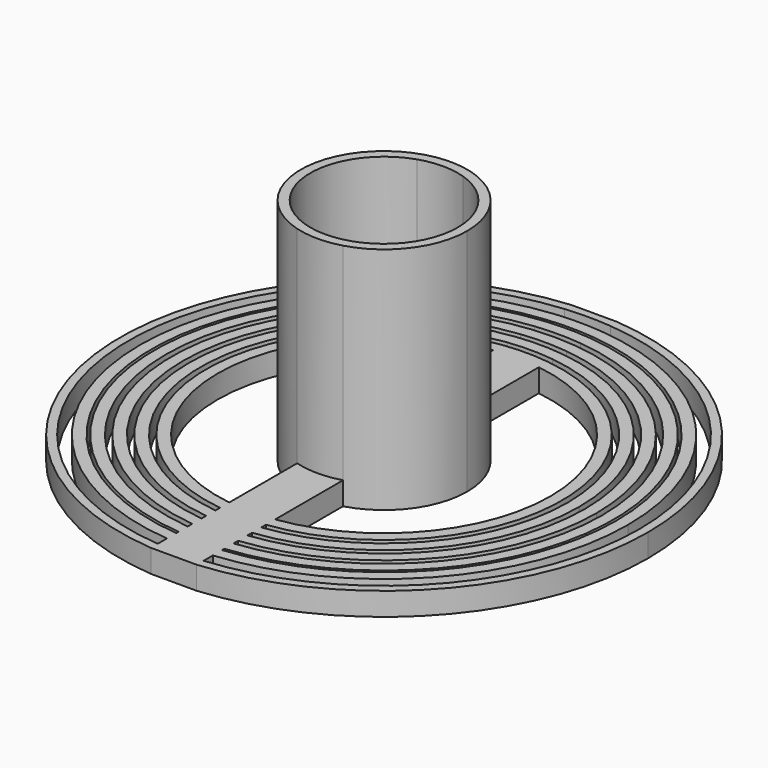
from build123d import *

# Parameters (mm, degrees)
F1_DEPTH = 40
F2_DEPTH = 4


with BuildPart() as f1:
    # F0 (on Top) → F1 (new body)
    with BuildSketch(Plane.XY):
        with BuildLine():
            ThreePointArc((4, 12.2115723803), (10.4048666498, 7.5406398933), (12.85, 0))
            ThreePointArc((12.85, 0), (10.4048666498, -7.5406398933), (4, -12.2115723803))
            Line((4, -12.2115723803), (4, -13.9373598648))
            ThreePointArc((4, -13.9373598648), (11.5812348219, -8.7249641833), (14.5, 0))
            ThreePointArc((14.5, 0), (11.5812348219, 8.7249641833), (4, 13.9373598648))
            Line((4, 13.9373598648), (4, 12.2115723803))
        make_face()
        with BuildLine():
            ThreePointArc((-4, 12.2115723803), (0, 12.85), (4, 12.2115723803))
            Line((4, 12.2115723803), (4, 13.9373598648))
            ThreePointArc((4, 13.9373598648), (0, 14.5), (-4, 13.9373598648))
            Line((-4, 13.9373598648), (-4, 12.2115723803))
        make_face()
        with BuildLine():
            Line((4, -13.9373598648), (4, -12.2115723803))
            ThreePointArc((4, -12.2115723803), (0, -12.85), (-4, -12.2115723803))
            Line((-4, -12.2115723803), (-4, -13.9373598648))
            ThreePointArc((-4, -13.9373598648), (0, -14.5), (4, -13.9373598648))
        make_face()
        with BuildLine():
            ThreePointArc((-4, -12.2115723803), (-12.85, 0), (-4, 12.2115723803))
            Line((-4, 12.2115723803), (-4, 13.9373598648))
            ThreePointArc((-4, 13.9373598648), (-14.5, 0), (-4, -13.9373598648))
            Line((-4, -13.9373598648), (-4, -12.2115723803))
        make_face()
    extrude(amount=F1_DEPTH)

    # F0 (on Top) → F2 (join)
    with BuildSketch(Plane.XY):
        with BuildLine():
            Line((4, -28.7228132327), (4, -13.9373598648))
            ThreePointArc((4, -13.9373598648), (0, -14.5), (-4, -13.9373598648))
            Line((-4, -13.9373598648), (-4, -28.7228132327))
            ThreePointArc((-4, -28.7228132327), (0, -29), (4, -28.7228132327))
        make_face()
        with BuildLine():
            ThreePointArc((-4, 40.3019850628), (0, 40.5), (4, 40.3019850628))
            Line((4, 40.3019850628), (4, 42.3113459961))
            ThreePointArc((4, 42.3113459961), (0, 42.5), (-4, 42.3113459961))
            Line((-4, 42.3113459961), (-4, 40.3019850628))
        make_face()
        with BuildLine():
            ThreePointArc((-4, -40.3019850628), (-40.5, 0), (-4, 40.3019850628))
            Line((-4, 40.3019850628), (-4, 42.3113459961))
            ThreePointArc((-4, 42.3113459961), (-42.5, 0), (-4, -42.3113459961))
            Line((-4, -42.3113459961), (-4, -40.3019850628))
        make_face()
        with BuildLine():
            Line((4, -42.3113459961), (4, -40.3019850628))
            ThreePointArc((4, -40.3019850628), (0, -40.5), (-4, -40.3019850628))
            Line((-4, -40.3019850628), (-4, -42.3113459961))
            ThreePointArc((-4, -42.3113459961), (0, -42.5), (4, -42.3113459961))
        make_face()
        with BuildLine():
            Line((4, 42.3113459961), (4, 40.3019850628))
            ThreePointArc((4, 40.3019850628), (30.0187441443, 27.1868534406), (40.5, 0))
            ThreePointArc((40.5, 0), (30.0187441443, -27.1868534406), (4, -40.3019850628))
            Line((4, -40.3019850628), (4, -42.3113459961))
            ThreePointArc((4, -42.3113459961), (31.434455618, -28.6028844699), (42.5, 0))
            ThreePointArc((42.5, 0), (31.434455618, 28.6028844699), (4, 42.3113459961))
        make_face()
        with BuildLine():
            ThreePointArc((-4, 37.7888872554), (0, 38), (4, 37.7888872554))
            Line((4, 37.7888872554), (4, 39.7994974843))
            ThreePointArc((4, 39.7994974843), (0, 40), (-4, 39.7994974843))
            Line((-4, 39.7994974843), (-4, 37.7888872554))
        make_face()
        with BuildLine():
            ThreePointArc((-4, -37.7888872554), (-38, 0), (-4, 37.7888872554))
            Line((-4, 37.7888872554), (-4, 39.7994974843))
            ThreePointArc((-4, 39.7994974843), (-40, 0), (-4, -39.7994974843))
            Line((-4, -39.7994974843), (-4, -37.7888872554))
        make_face()
        with BuildLine():
            Line((4, -39.7994974843), (4, -37.7888872554))
            ThreePointArc((4, -37.7888872554), (0, -38), (-4, -37.7888872554))
            Line((-4, -37.7888872554), (-4, -39.7994974843))
            ThreePointArc((-4, -39.7994974843), (0, -40), (4, -39.7994974843))
        make_face()
        with BuildLine():
            Line((4, 39.7994974843), (4, 37.7888872554))
            ThreePointArc((4, 37.7888872554), (28.2488937837, 25.4165300543), (38, 0))
            ThreePointArc((38, 0), (28.2488937837, -25.4165300543), (4, -37.7888872554))
            Line((4, -37.7888872554), (4, -39.7994974843))
            ThreePointArc((4, -39.7994974843), (29.6647939484, -26.83281573), (40, 0))
            ThreePointArc((40, 0), (29.6647939484, 26.83281573), (4, 39.7994974843))
        make_face()
        with BuildLine():
            Line((4, -40.3019850628), (4, -39.7994974843))
            ThreePointArc((4, -39.7994974843), (0, -40), (-4, -39.7994974843))
            Line((-4, -39.7994974843), (-4, -40.3019850628))
            ThreePointArc((-4, -40.3019850628), (0, -40.5), (4, -40.3019850628))
        make_face()
        with BuildLine():
            Line((4, -44.3198601081), (4, -42.3113459961))
            ThreePointArc((4, -42.3113459961), (0, -42.5), (-4, -42.3113459961))
            Line((-4, -42.3113459961), (-4, -44.3198601081))
            ThreePointArc((-4, -44.3198601081), (0, -44.5), (4, -44.3198601081))
        make_face()
        with BuildLine():
            ThreePointArc((-4, -44.3198601081), (-44.5, 0), (-4, 44.3198601081))
            Line((-4, 44.3198601081), (-4, 45.8257569496))
            ThreePointArc((-4, 45.8257569496), (-46, 0), (-4, -45.8257569496))
            Line((-4, -45.8257569496), (-4, -44.3198601081))
        make_face()
        with BuildLine():
            Line((4, 45.8257569496), (4, 44.3198601081))
            ThreePointArc((4, 44.3198601081), (32.8500380517, 30.0187441443), (44.5, 0))
            ThreePointArc((44.5, 0), (32.8500380517, -30.0187441443), (4, -44.3198601081))
            Line((4, -44.3198601081), (4, -45.8257569496))
            ThreePointArc((4, -45.8257569496), (33.9116499156, -31.0805405358), (46, 0))
            ThreePointArc((46, 0), (33.9116499156, 31.0805405358), (4, 45.8257569496))
        make_face()
        with BuildLine():
            ThreePointArc((-4, 44.3198601081), (0, 44.5), (4, 44.3198601081))
            Line((4, 44.3198601081), (4, 45.8257569496))
            Line((4, 45.8257569496), (-4, 45.8257569496))
            Line((-4, 45.8257569496), (-4, 44.3198601081))
        make_face()
        with BuildLine():
            Line((4, -45.8257569496), (4, -44.3198601081))
            ThreePointArc((4, -44.3198601081), (0, -44.5), (-4, -44.3198601081))
            Line((-4, -44.3198601081), (-4, -45.8257569496))
            Line((-4, -45.8257569496), (4, -45.8257569496))
        make_face()
        with BuildLine():
            ThreePointArc((-4, -34.7706773014), (-35, 0), (-4, 34.7706773014))
            Line((-4, 34.7706773014), (-4, 36.7831483155))
            ThreePointArc((-4, 36.7831483155), (-37, 0), (-4, -36.7831483155))
            Line((-4, -36.7831483155), (-4, -34.7706773014))
        make_face()
        with BuildLine():
            ThreePointArc((-4, -31.7490157328), (-32, 0), (-4, 31.7490157328))
            Line((-4, 31.7490157328), (-4, 33.7638860323))
            ThreePointArc((-4, 33.7638860323), (-34, 0), (-4, -33.7638860323))
            Line((-4, -33.7638860323), (-4, -31.7490157328))
        make_face()
        with BuildLine():
            ThreePointArc((-4, -28.7228132327), (-29, 0), (-4, 28.7228132327))
            Line((-4, 28.7228132327), (-4, 30.7408522979))
            ThreePointArc((-4, 30.7408522979), (-31, 0), (-4, -30.7408522979))
            Line((-4, -30.7408522979), (-4, -28.7228132327))
        make_face()
        with BuildLine():
            Line((4, 36.7831483155), (4, 34.7706773014))
            ThreePointArc((4, 34.7706773014), (26.1247009552, 23.2916293977), (35, 0))
            ThreePointArc((35, 0), (26.1247009552, -23.2916293977), (4, -34.7706773014))
            Line((4, -34.7706773014), (4, -36.7831483155))
            ThreePointArc((4, -36.7831483155), (27.5408787078, -24.7082982012), (37, 0))
            ThreePointArc((37, 0), (27.5408787078, 24.7082982012), (4, 36.7831483155))
        make_face()
        with BuildLine():
            Line((4, 33.7638860323), (4, 31.7490157328))
            ThreePointArc((4, 31.7490157328), (24, 21.1660104885), (32, 0))
            ThreePointArc((32, 0), (24, -21.1660104885), (4, -31.7490157328))
            Line((4, -31.7490157328), (4, -33.7638860323))
            ThreePointArc((4, -33.7638860323), (25.4165300543, -22.5831795813), (34, 0))
            ThreePointArc((34, 0), (25.4165300543, 22.5831795813), (4, 33.7638860323))
        make_face()
        with BuildLine():
            Line((4, 30.7408522979), (4, 28.7228132327))
            ThreePointArc((4, 28.7228132327), (21.8746428542, 19.0394327647), (29, 0))
            ThreePointArc((29, 0), (21.8746428542, -19.0394327647), (4, -28.7228132327))
            Line((4, -28.7228132327), (4, -30.7408522979))
            ThreePointArc((4, -30.7408522979), (23.2916293977, -20.4572725455), (31, 0))
            ThreePointArc((31, 0), (23.2916293977, 20.4572725455), (4, 30.7408522979))
        make_face()
        with BuildLine():
            ThreePointArc((-4, 28.7228132327), (0, 29), (4, 28.7228132327))
            Line((4, 28.7228132327), (4, 30.7408522979))
            ThreePointArc((4, 30.7408522979), (0, 31), (-4, 30.7408522979))
            Line((-4, 30.7408522979), (-4, 28.7228132327))
        make_face()
        with BuildLine():
            ThreePointArc((-4, 31.7490157328), (0, 32), (4, 31.7490157328))
            Line((4, 31.7490157328), (4, 33.7638860323))
            ThreePointArc((4, 33.7638860323), (0, 34), (-4, 33.7638860323))
            Line((-4, 33.7638860323), (-4, 31.7490157328))
        make_face()
        with BuildLine():
            ThreePointArc((-4, 34.7706773014), (0, 35), (4, 34.7706773014))
            Line((4, 34.7706773014), (4, 36.7831483155))
            ThreePointArc((4, 36.7831483155), (0, 37), (-4, 36.7831483155))
            Line((-4, 36.7831483155), (-4, 34.7706773014))
        make_face()
        with BuildLine():
            Line((4, -30.7408522979), (4, -28.7228132327))
            ThreePointArc((4, -28.7228132327), (0, -29), (-4, -28.7228132327))
            Line((-4, -28.7228132327), (-4, -30.7408522979))
            ThreePointArc((-4, -30.7408522979), (0, -31), (4, -30.7408522979))
        make_face()
        with BuildLine():
            Line((4, -33.7638860323), (4, -31.7490157328))
            ThreePointArc((4, -31.7490157328), (0, -32), (-4, -31.7490157328))
            Line((-4, -31.7490157328), (-4, -33.7638860323))
            ThreePointArc((-4, -33.7638860323), (0, -34), (4, -33.7638860323))
        make_face()
        with BuildLine():
            Line((4, -36.7831483155), (4, -34.7706773014))
            ThreePointArc((4, -34.7706773014), (0, -35), (-4, -34.7706773014))
            Line((-4, -34.7706773014), (-4, -36.7831483155))
            ThreePointArc((-4, -36.7831483155), (0, -37), (4, -36.7831483155))
        make_face()
        with BuildLine():
            Line((4, -31.7490157328), (4, -30.7408522979))
            ThreePointArc((4, -30.7408522979), (0, -31), (-4, -30.7408522979))
            Line((-4, -30.7408522979), (-4, -31.7490157328))
            ThreePointArc((-4, -31.7490157328), (0, -32), (4, -31.7490157328))
        make_face()
        with BuildLine():
            Line((4, -34.7706773014), (4, -33.7638860323))
            ThreePointArc((4, -33.7638860323), (0, -34), (-4, -33.7638860323))
            Line((-4, -33.7638860323), (-4, -34.7706773014))
            ThreePointArc((-4, -34.7706773014), (0, -35), (4, -34.7706773014))
        make_face()
        with BuildLine():
            Line((4, -37.7888872554), (4, -36.7831483155))
            ThreePointArc((4, -36.7831483155), (0, -37), (-4, -36.7831483155))
            Line((-4, -36.7831483155), (-4, -37.7888872554))
            ThreePointArc((-4, -37.7888872554), (0, -38), (4, -37.7888872554))
        make_face()
        with BuildLine():
            ThreePointArc((-4, 13.9373598648), (0, 14.5), (4, 13.9373598648))
            Line((4, 13.9373598648), (4, 28.7228132327))
            ThreePointArc((4, 28.7228132327), (0, 29), (-4, 28.7228132327))
            Line((-4, 28.7228132327), (-4, 13.9373598648))
        make_face()
    extrude(amount=F2_DEPTH)


solid = f1.part
